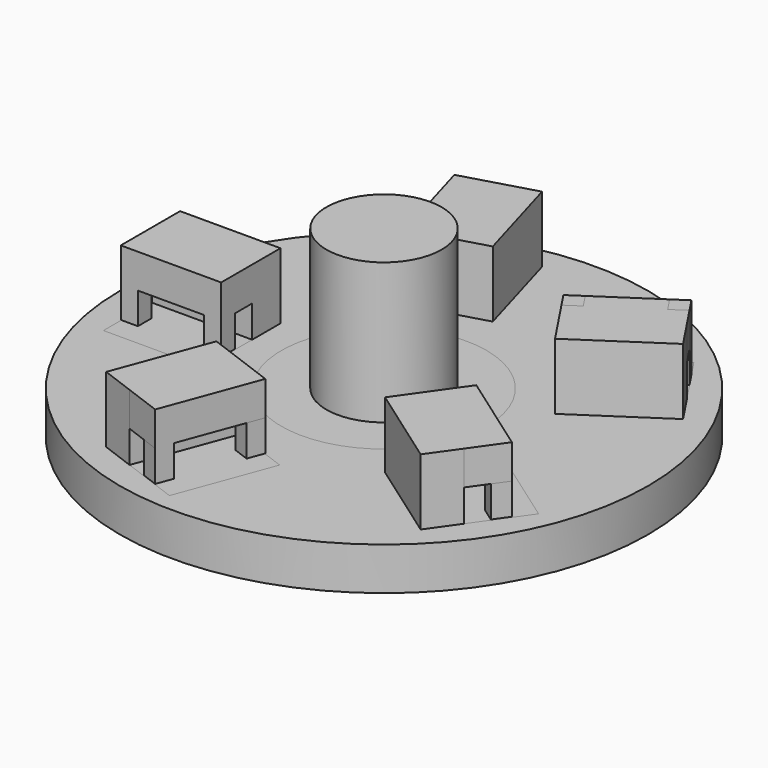
from build123d import *

# Parameters (mm, degrees)
F0_R      = 23.155
F0_R_2    = 9
F1_DEPTH  = 3.75
F0_R_3    = 6.3
F2_DEPTH  = 5.75
F3_DEPTH  = 5.8
F4_DEPTH  = 3.75
F5_W      = 8.8
F5_H      = 3
F6_DEPTH  = 3.4
F0_W      = 8.8
F0_H      = 3.1
F7_DEPTH  = 5.8
F8_W      = 8.8
F8_H      = 3
F9_DEPTH  = 3.4
F10_W     = 8.8
F10_H     = 3
F11_DEPTH = 3.4
F12_DEPTH = 3.75
F13_W     = 8.8
F13_H     = 3
F14_DEPTH = 3.4
F15_W     = 8.8
F15_H     = 3
F16_DEPTH = 3.4
F0_R_4    = 5.05
F17_DEPTH = 3.75
F18_DEPTH = 3.75
F19_DEPTH = 10.35
F20_R     = 5.05
F21_DEPTH = 2
F22_DEPTH = 3.75
F0_H_2    = 5.3
F24_DEPTH = 5.75
F26_DEPTH = 5.75
F28_DEPTH = 5.75
F29_W     = 1.5
F29_H     = 1.5
F30_DEPTH = 5.75
F32_DEPTH = 5.75


with BuildPart() as f1:
    # F0 (on Top) → F1 (new body)
    with BuildSketch(Plane.XY):
        Circle(F0_R)
        Polygon((-6.3585940178, -10.415183582), (-3.4519187473, -11.4927915217), (1.5175583281, -13.3351534831), (-1.5414577587, -21.5863607027), (-6.5109348342, -19.7439987413), (-9.4176101047, -18.6663908016), align=None, mode=Mode.SUBTRACT)
        Polygon((-11.556814377, 3.1), (-11.556814377, 0), (-11.556814377, -5.3), (-20.356814377, -5.3), (-20.356814377, 0), (-20.356814377, 3.1), align=None, mode=Mode.SUBTRACT)
        Polygon((7.8428340275, -9.6869680469), (9.6328495933, -7.1559911062), (12.6931987865, -2.8288369818), (19.8779075213, -7.9101714912), (16.8175583281, -12.2373256156), (15.0275427623, -14.7683025563), align=None, mode=Mode.SUBTRACT)
        Polygon((-0.3715475496, 12.383882616), (-3.3496206529, 11.5230222373), (-6.8080281277, 10.5233134105), (-8.4411649907, 10.0512286867), (-10.8848976785, 18.5051136251), (-9.2517608154, 18.9771983489), (-5.7933533406, 19.9769071757), (-2.8152802374, 20.8377675543), align=None, mode=Mode.SUBTRACT)
        Circle(F0_R_2, mode=Mode.SUBTRACT)
        Polygon((11.5002745688, 4.3658506272), (9.7842418084, 6.9475616035), (6.8503793471, 11.361454563), (14.1791072799, 16.2327733667), (17.1129697412, 11.8188804072), (18.8290025016, 9.2371694308), align=None, mode=Mode.SUBTRACT)
    extrude(amount=-F1_DEPTH)

    # F0 (on Top) → F4 (join)
    with BuildSketch(Plane.XY):
        Polygon((-5.7933533406, 19.9769071757), (-3.3496206529, 11.5230222373), (-0.3715475496, 12.383882616), (-2.8152802374, 20.8377675543), align=None)
    extrude(amount=-F4_DEPTH)


with BuildPart() as f2:
    # F0 (on Top) → F2 (new body)
    with BuildSketch(Plane.XY):
        Circle(F0_R_2)
        Circle(F0_R_3, mode=Mode.SUBTRACT)
    extrude(amount=-F2_DEPTH)

    # F0 (on Top) → F17 (join)
    with BuildSketch(Plane.XY):
        Circle(F0_R_3)
        Circle(F0_R_4, mode=Mode.SUBTRACT)
    extrude(amount=-F17_DEPTH)

    # F0 (on Top) → F18 (join)
    with BuildSketch(Plane.XY):
        Circle(F0_R_4)
        with BuildLine():
            Line((2.6031833563, 2.447395), (2.6031833563, -2.447395))
            ThreePointArc((2.6031833563, -2.447395), (1.4180570261, -3.2795457221), (0, -3.5729967636))
            ThreePointArc((0, -3.5729967636), (-1.4180570261, -3.2795457221), (-2.6031833563, -2.447395))
            Line((-2.6031833563, -2.447395), (-2.6031833563, 2.447395))
            ThreePointArc((-2.6031833563, 2.447395), (-1.4180570261, 3.2795457221), (0, 3.5729967636))
            ThreePointArc((0, 3.5729967636), (1.4180570261, 3.2795457221), (2.6031833563, 2.447395))
        make_face(mode=Mode.SUBTRACT)
    extrude(amount=-F18_DEPTH)

    # F0 (on Top) → F19 (join)
    with BuildSketch(Plane.XY):
        Circle(F0_R_4)
        with BuildLine():
            Line((2.6031833563, 2.447395), (2.6031833563, -2.447395))
            ThreePointArc((2.6031833563, -2.447395), (1.4180570261, -3.2795457221), (0, -3.5729967636))
            ThreePointArc((0, -3.5729967636), (-1.4180570261, -3.2795457221), (-2.6031833563, -2.447395))
            Line((-2.6031833563, -2.447395), (-2.6031833563, 2.447395))
            ThreePointArc((-2.6031833563, 2.447395), (-1.4180570261, 3.2795457221), (0, 3.5729967636))
            ThreePointArc((0, 3.5729967636), (1.4180570261, 3.2795457221), (2.6031833563, 2.447395))
        make_face(mode=Mode.SUBTRACT)
    extrude(amount=F19_DEPTH)

    # F20 (on face) → F21 (join)
    with BuildSketch(Plane.XY.offset(10.35)):
        Circle(F20_R)
        with BuildLine():
            ThreePointArc((-2.6031833563, 2.447395), (0, 3.5729967636), (2.6031833563, 2.447395))
            Line((2.6031833563, 2.447395), (2.6031833563, -2.447395))
            ThreePointArc((2.6031833563, -2.447395), (0, -3.5729967636), (-2.6031833563, -2.447395))
            Line((-2.6031833563, -2.447395), (-2.6031833563, 2.447395))
        make_face(mode=Mode.SUBTRACT)
        with BuildLine():
            Line((2.6031833563, -2.447395), (2.6031833563, 2.447395))
            ThreePointArc((2.6031833563, 2.447395), (0, 3.5729967636), (-2.6031833563, 2.447395))
            Line((-2.6031833563, 2.447395), (-2.6031833563, -2.447395))
            ThreePointArc((-2.6031833563, -2.447395), (0, -3.5729967636), (2.6031833563, -2.447395))
        make_face()
    extrude(amount=F21_DEPTH)


with BuildPart() as f3:
    # F0 (on Top) → F3 (new body)
    with BuildSketch(Plane.XY):
        Polygon((-5.7933533406, 19.9769071757), (-3.3496206529, 11.5230222373), (-0.3715475496, 12.383882616), (-2.8152802374, 20.8377675543), align=None)
    extrude(amount=F3_DEPTH)

    # F5 (on face) → F6 (join)
    with BuildSketch(Plane(origin=(-0.0172616326, -0.0049897551, 0), x_dir=(0.2776968963, -0.960668743, 0), z_dir=(-0.960668743, -0.2776968963, 0))):
        with Locations((-16.3999865474, 4.3)):
            Rectangle(F5_W, F5_H)
    extrude(amount=F6_DEPTH)

    # F31 (on face) → F32 (join)
    with BuildSketch(Plane.XY.offset(5.8)):
        Polygon((-5.5914366091, 12.4364012488), (-7.0324397236, 12.0198559043), (-6.6158943791, 10.5788527898), (-5.1748912646, 10.9953981343), align=None)
        Polygon((-9.0596270668, 19.0327377281), (-8.6430817223, 17.5917346136), (-7.2020786078, 18.0082799581), (-7.6186239523, 19.4492830726), align=None)
    extrude(amount=-F32_DEPTH)


with BuildPart() as f7:
    # F0 (on Top) → F7 (new body)
    with BuildSketch(Plane.XY):
        with Locations((-15.956814377, 1.55)):
            Rectangle(F0_W, F0_H)
    extrude(amount=F7_DEPTH)

    # F8 (on face) → F9 (join)
    with BuildSketch(Plane.XZ):
        with Locations((-15.956814377, 4.3)):
            Rectangle(F8_W, F8_H)
    extrude(amount=F9_DEPTH)

    # F29 (on face) → F30 (join)
    with BuildSketch(Plane.XY.offset(5.8)):
        with Locations((-19.606814377, -2.65)):
            Rectangle(F29_W, F29_H)
        with Locations((-12.306814377, -2.65)):
            Rectangle(F29_W, F29_H)
    extrude(amount=-F30_DEPTH)


with BuildPart() as f7b:
    # F0 (on Top) → F7, piece 2 (new body)
    with BuildSketch(Plane.XY):
        Polygon((17.1129697412, 11.8188804072), (9.7842418084, 6.9475616035), (11.5002745688, 4.3658506272), (18.8290025016, 9.2371694308), align=None)
    extrude(amount=F7_DEPTH)

    # F15 (on face) → F16 (join)
    with BuildSketch(Plane(origin=(-0.2047304888, 0.308009825, 0), x_dir=(-0.8328099924, -0.553558955, 0), z_dir=(-0.553558955, 0.8328099924, 0))):
        with Locations((-16.3942992865, 4.3)):
            Rectangle(F15_W, F15_H)
    extrude(amount=F16_DEPTH)


with BuildPart() as f7c:
    # F0 (on Top) → F7, piece 3 (new body)
    with BuildSketch(Plane.XY):
        Polygon((16.8175583281, -12.2373256156), (9.6328495933, -7.1559911062), (7.8428340275, -9.6869680469), (15.0275427623, -14.7683025563), align=None)
    extrude(amount=F7_DEPTH)

    # F13 (on face) → F14 (join)
    with BuildSketch(Plane(origin=(-0.1618087946, -0.2287881378, 0), x_dir=(-0.8164441744, 0.5774243761, 0), z_dir=(0.5774243761, 0.8164441744, 0))):
        with Locations((-16.3967276331, 4.3)):
            Rectangle(F13_W, F13_H)
    extrude(amount=F14_DEPTH)

    # F25 (on face) → F26 (join)
    with BuildSketch(Plane.XY.offset(5.8)):
        Polygon((16.689998381, -9.8199451201), (17.9146646427, -10.6860816842), (18.7808012068, -9.4614154226), (17.5561349451, -8.5952788585), align=None)
        Polygon((11.9546221695, -6.4708837389), (12.8207587336, -5.2462174773), (11.596092472, -4.3800809132), (10.7299559079, -5.6047471748), align=None)
    extrude(amount=-F26_DEPTH)


with BuildPart() as f7d:
    # F0 (on Top) → F7, piece 4 (new body)
    with BuildSketch(Plane.XY):
        Polygon((-6.5109348342, -19.7439987413), (-3.4519187473, -11.4927915217), (-6.3585940178, -10.415183582), (-9.4176101047, -18.6663908016), align=None)
    extrude(amount=F7_DEPTH)

    # F10 (on face) → F11 (join)
    with BuildSketch(Plane(origin=(0.7111271892, -0.2636401503, 0), x_dir=(0.3476154644, 0.937637184, 0), z_dir=(0.937637184, -0.3476154644, 0))):
        with Locations((-16.3760090177, 4.3)):
            Rectangle(F10_W, F10_H)
    extrude(amount=F11_DEPTH)

    # F27 (on face) → F28 (join)
    with BuildSketch(Plane.XY.offset(5.8)):
        Polygon((-4.2080009878, -18.9980123476), (-4.7294241845, -20.4044681237), (-3.3229684084, -20.9258913203), (-2.8015452118, -19.5194355443), align=None)
        Polygon((-2.1918312942, -13.5597166802), (-0.7853755182, -14.0811398768), (-0.2639523216, -12.6746841007), (-1.6704080976, -12.1532609041), align=None)
    extrude(amount=-F28_DEPTH)


with BuildPart() as f12:
    # F0 (on Top) → F12 (new body)
    with BuildSketch(Plane.XY):
        with Locations((-15.956814377, 1.55)):
            Rectangle(F0_W, F0_H)
    extrude(amount=-F12_DEPTH)


with BuildPart() as f12b:
    # F0 (on Top) → F12, piece 2 (new body)
    with BuildSketch(Plane.XY):
        Polygon((-6.5109348342, -19.7439987413), (-3.4519187473, -11.4927915217), (-6.3585940178, -10.415183582), (-9.4176101047, -18.6663908016), align=None)
    extrude(amount=-F12_DEPTH)


with BuildPart() as f12c:
    # F0 (on Top) → F12, piece 3 (new body)
    with BuildSketch(Plane.XY):
        Polygon((17.1129697412, 11.8188804072), (9.7842418084, 6.9475616035), (11.5002745688, 4.3658506272), (18.8290025016, 9.2371694308), align=None)
    extrude(amount=-F12_DEPTH)


with BuildPart() as f12d:
    # F0 (on Top) → F12, piece 4 (new body)
    with BuildSketch(Plane.XY):
        Polygon((16.8175583281, -12.2373256156), (9.6328495933, -7.1559911062), (7.8428340275, -9.6869680469), (15.0275427623, -14.7683025563), align=None)
    extrude(amount=-F12_DEPTH)


with BuildPart() as f22:
    # F0 (on Top) → F22 (new body)
    with BuildSketch(Plane.XY):
        Polygon((-8.4411649907, 10.0512286867), (-6.8080281277, 10.5233134105), (-9.2517608154, 18.9771983489), (-10.8848976785, 18.5051136251), align=None)
        Polygon((-6.8080281277, 10.5233134105), (-3.3496206529, 11.5230222373), (-5.7933533406, 19.9769071757), (-9.2517608154, 18.9771983489), align=None)
    extrude(amount=-F22_DEPTH)


with BuildPart() as f22b:
    # F0 (on Top) → F22, piece 2 (new body)
    with BuildSketch(Plane.XY):
        with Locations((-15.956814377, -2.65)):
            Rectangle(F0_W, F0_H_2)
    extrude(amount=-F22_DEPTH)


with BuildPart() as f22c:
    # F0 (on Top) → F22, piece 3 (new body)
    with BuildSketch(Plane.XY):
        Polygon((1.5175583281, -13.3351534831), (-3.4519187473, -11.4927915217), (-6.5109348342, -19.7439987413), (-1.5414577587, -21.5863607027), align=None)
    extrude(amount=-F22_DEPTH)


with BuildPart() as f22d:
    # F0 (on Top) → F22, piece 4 (new body)
    with BuildSketch(Plane.XY):
        Polygon((12.6931987865, -2.8288369818), (9.6328495933, -7.1559911062), (16.8175583281, -12.2373256156), (19.8779075213, -7.9101714912), align=None)
    extrude(amount=-F22_DEPTH)


with BuildPart() as f22e:
    # F0 (on Top) → F22, piece 5 (new body)
    with BuildSketch(Plane.XY):
        Polygon((6.8503793471, 11.361454563), (9.7842418084, 6.9475616035), (17.1129697412, 11.8188804072), (14.1791072799, 16.2327733667), align=None)
    extrude(amount=-F22_DEPTH)


with BuildPart() as f24:
    # F23 (on face) → F24 (new body)
    with BuildSketch(Plane.XY.offset(5.8)):
        Polygon((14.8119927383, 12.5708809602), (16.0612077268, 13.4012193926), (15.2308692944, 14.6504343812), (13.9816543058, 13.8200959488), align=None)
    extrude(amount=-F24_DEPTH)


with BuildPart() as f24b:
    # F23 (on face) → F24, piece 2 (new body)
    with BuildSketch(Plane.XY.offset(5.8)):
        Polygon((9.9816947825, 9.3602390214), (9.1513563501, 10.60945401), (7.9021413615, 9.7791155775), (8.732479794, 8.529900589), align=None)
    extrude(amount=-F24_DEPTH)


solid = Compound([f1.part, f2.part, f3.part, f7.part, f7b.part, f7c.part, f7d.part, f12.part, f12b.part, f12c.part, f12d.part, f22.part, f22b.part, f22c.part, f22d.part, f22e.part, f24.part, f24b.part])
